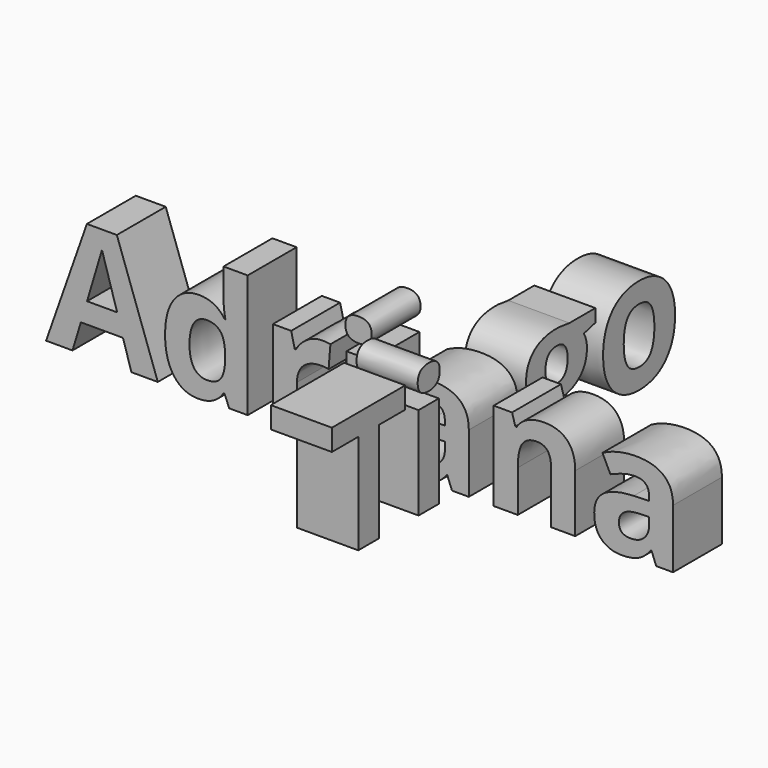
from build123d import *

# Parameters (mm, degrees)
F0_TEXT_SIZE = 39.7444405179
F1_DEPTH     = 15
F2_TEXT_SIZE = 41.7329034665
F3_DEPTH     = 15


# Not quite as in the source:
# - Text() gives the source's letters only with a copy of the font that has no kerning and outlines rounded to 1/6400 em; it was checked with that copy


with BuildPart() as f1:
    # F0 (on Front) → F1 (new body)
    with BuildSketch(Plane.XZ):
        with Locations((-86.0893763602, 0)):
            Text('Adriana', F0_TEXT_SIZE, font='Open Sans', font_style=FontStyle.BOLD, text_align=(TextAlign.LEFT, TextAlign.BOTTOM))
    extrude(amount=F1_DEPTH)


with BuildPart() as f3:
    # F2 (on Right) → F3 (new body)
    with BuildSketch(Plane.YZ):
        with Locations((-54.5017290142, 0)):
            Text('Ti  go', F2_TEXT_SIZE, font='Open Sans', font_style=FontStyle.BOLD, text_align=(TextAlign.LEFT, TextAlign.BOTTOM))
    extrude(amount=F3_DEPTH)


solid = Compound([f1.part, f3.part])
